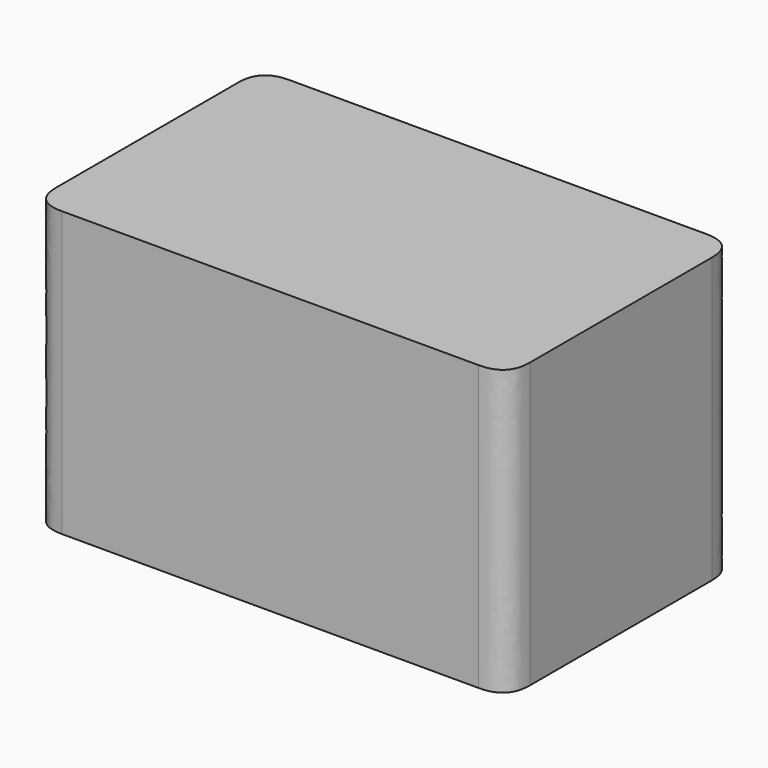
from build123d import *

# Parameters (mm, degrees)
F0_W        = 49.9999988824
F0_H        = 29.9999988824
F0_W_2      = 45.8000008941
F0_H_2      = 25.8000008941
F0_W_3      = 45.0000008941
F0_H_3      = 25.0000008941
F0_W_4      = 40
F0_H_4      = 20
F1_DEPTH    = 30
F2_DEPTH    = 25
F3_T1_DEPTH = 45


# Not quite as in the source:
# - a fillet or chamfer that OpenCascade refuses, or shapes differently, is made with other operations: its cross-section is extruded or revolved along the edge and cut away or added


with BuildPart() as f1:
    # F0 (on Top) → F1 (new body)
    with BuildSketch(Plane.XY):
        Rectangle(F0_W, F0_H)
        Rectangle(F0_W_2, F0_H_2, mode=Mode.SUBTRACT)
        Rectangle(F0_W_2, F0_H_2)
        Rectangle(F0_W_3, F0_H_3, mode=Mode.SUBTRACT)
        Rectangle(F0_W_3, F0_H_3)
        Rectangle(F0_W_4, F0_H_4, mode=Mode.SUBTRACT)
        Rectangle(F0_W_4, F0_H_4)
    extrude(amount=F1_DEPTH)

    # F0 (on Top) → F2 (cut)
    with BuildSketch(Plane.XY):
        Rectangle(F0_W_2, F0_H_2)
        Rectangle(F0_W_3, F0_H_3, mode=Mode.SUBTRACT)
        Rectangle(F0_W_3, F0_H_3)
        Rectangle(F0_W_4, F0_H_4, mode=Mode.SUBTRACT)
        Rectangle(F0_W_4, F0_H_4)
    extrude(amount=F2_DEPTH, mode=Mode.SUBTRACT)

    # F3: fillet of radius 3 on 4 edges, made by hand

    # F3_s2 → F3_t1 (cut)
    with BuildSketch(Plane.XY.offset(-7.5)):
        with BuildLine():
            add(Edge.make_bspline(
                [(-21.9999994412, -14.9999994412), (-24.9999994412, -14.9999994412), (-24.9999994412, -11.9999994412)],
                knots=[0, 0, 0, 1, 1, 1], degree=2, weights=[1, 1, 1]))
            Line((-24.9999994412, -11.9999994412), (-24.9999994412, -14.9999994412))
            Line((-24.9999994412, -14.9999994412), (-21.9999994412, -14.9999994412))
        make_face()
        with BuildLine():
            add(Edge.make_bspline(
                [(-24.9999994412, 11.9999994412), (-24.9999994412, 14.9999994412), (-21.9999994412, 14.9999994412)],
                knots=[0, 0, 0, 1, 1, 1], degree=2, weights=[1, 1, 1]))
            Line((-21.9999994412, 14.9999994412), (-24.9999994412, 14.9999994412))
            Line((-24.9999994412, 14.9999994412), (-24.9999994412, 11.9999994412))
        make_face()
        with BuildLine():
            add(Edge.make_bspline(
                [(21.9999994412, -14.9999994412), (24.9999994412, -14.9999994412), (24.9999994412, -11.9999994412)],
                knots=[0, 0, 0, 1, 1, 1], degree=2, weights=[1, 1, 1]))
            Line((24.9999994412, -11.9999994412), (24.9999994412, -14.9999994412))
            Line((24.9999994412, -14.9999994412), (21.9999994412, -14.9999994412))
        make_face()
        with BuildLine():
            add(Edge.make_bspline(
                [(24.9999994412, 11.9999994412), (24.9999994412, 14.9999994412), (21.9999994412, 14.9999994412)],
                knots=[0, 0, 0, 1, 1, 1], degree=2, weights=[1, 1, 1]))
            Line((21.9999994412, 14.9999994412), (24.9999994412, 14.9999994412))
            Line((24.9999994412, 14.9999994412), (24.9999994412, 11.9999994412))
        make_face()
    extrude(amount=F3_T1_DEPTH, mode=Mode.SUBTRACT)


solid = f1.part
